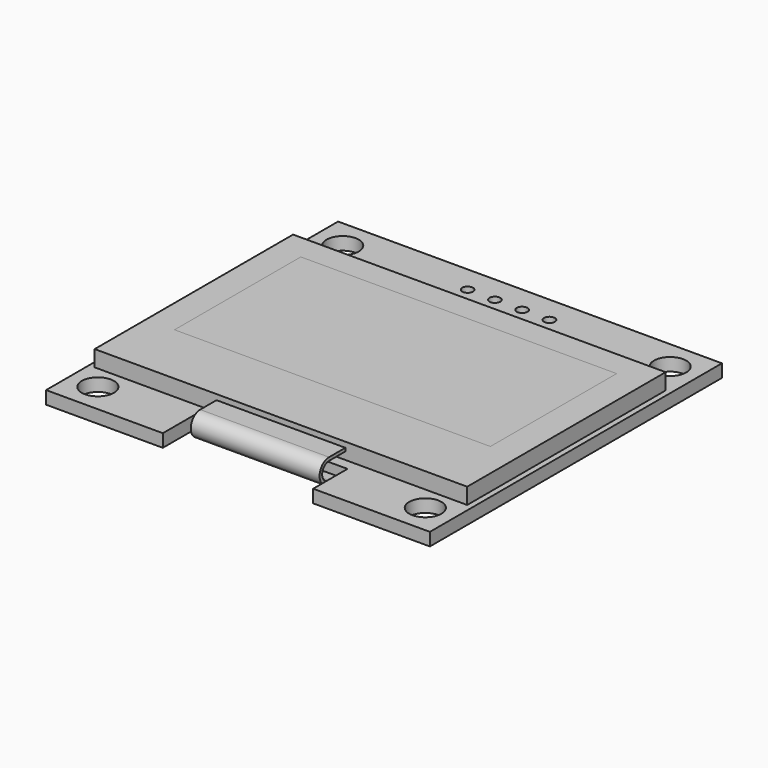
from build123d import *

# Parameters (mm, degrees)
F0_R     = 1.5
F0_R_2   = 0.5
F1_DEPTH = 1.2
F2_W     = 34.7
F2_H     = 23.1
F2_W_2   = 29.42
F2_H_2   = 14.7
F3_DEPTH = 1.5
F4_DEPTH = 1.5
F6_DEPTH = 6
F7_W     = 0.762
F7_H     = 1.524
F7_W_2   = 1.65
F7_H_2   = 3
F7_W_3   = 1.524
F7_H_3   = 0.762
F8_DEPTH = 0.9


with BuildPart() as f1:
    # F0 (on Top) → F1 (new body)
    with BuildSketch(Plane.XY):
        Polygon((17.875, 0), (17.875, 34), (-17.875, 34), (-17.875, 0), (-7, 0), (-7, 4), (7, 4), (7, 0), align=None)
        with Locations((-15.25, 2.75)):
            Circle(F0_R, mode=Mode.SUBTRACT)
        with Locations((15.25, 2.75)):
            Circle(F0_R, mode=Mode.SUBTRACT)
        with Locations((-15.25, 31.25)):
            Circle(F0_R, mode=Mode.SUBTRACT)
        with Locations((-3.81, 31.5)):
            Circle(F0_R_2, mode=Mode.SUBTRACT)
        with Locations((-1.27, 31.5)):
            Circle(F0_R_2, mode=Mode.SUBTRACT)
        with Locations((1.27, 31.5)):
            Circle(F0_R_2, mode=Mode.SUBTRACT)
        with Locations((3.81, 31.5)):
            Circle(F0_R_2, mode=Mode.SUBTRACT)
        with Locations((15.25, 31.25)):
            Circle(F0_R, mode=Mode.SUBTRACT)
    extrude(amount=-F1_DEPTH)

    # F7 (on face) → F8 (join)
    with BuildSketch(Plane(origin=(0, 0, -1.2), x_dir=(1, 0, 0), z_dir=(0, 0, -1))):
        with Locations((15.194, -16.962)):
            Rectangle(F7_W, F7_H)
        with Locations((13.1723636364, -16.962)):
            Rectangle(F7_W, F7_H)
        with Locations((11.1507272727, -16.962)):
            Rectangle(F7_W, F7_H)
        with Locations((9.1290909091, -16.962)):
            Rectangle(F7_W, F7_H)
        with Locations((7.1074545455, -16.962)):
            Rectangle(F7_W, F7_H)
        with Locations((5.0858181818, -16.962)):
            Rectangle(F7_W, F7_H)
        with Locations((3.0641818182, -16.962)):
            Rectangle(F7_W, F7_H)
        with Locations((1.0425454545, -16.962)):
            Rectangle(F7_W, F7_H)
        with Locations((-0.9790909091, -16.962)):
            Rectangle(F7_W, F7_H)
        with Locations((-3.0007272727, -16.962)):
            Rectangle(F7_W, F7_H)
        with Locations((-5.0223636364, -16.962)):
            Rectangle(F7_W, F7_H)
        with Locations((-7.044, -16.962)):
            Rectangle(F7_W, F7_H)
        with Locations((-10.082, -16.962)):
            Rectangle(F7_W, F7_H)
        with Locations((-12.544, -16.962)):
            Rectangle(F7_W, F7_H)
        with Locations((-8.15, -22.5)):
            Rectangle(F7_W_2, F7_H_2)
        with Locations((-7.413, -26.219)):
            Rectangle(F7_W_3, F7_H_3)
        with Locations((2.613, -23.219)):
            Rectangle(F7_W_3, F7_H_3)
    extrude(amount=F8_DEPTH)


with BuildPart() as f3:
    # F2 (on Top) → F3 (new body)
    with BuildSketch(Plane.XY):
        with Locations((0, 16.55)):
            Rectangle(F2_W, F2_H)
        with Locations((0, 18.35)):
            Rectangle(F2_W_2, F2_H_2, mode=Mode.SUBTRACT)
    extrude(amount=F3_DEPTH)

    # F5 (on Right) → F6 (join, symmetric)
    with BuildSketch(Plane.YZ):
        with BuildLine():
            Line((5, 1), (3.1, 1))
            ThreePointArc((3.1, 1), (2, -0.1), (3.1, -1.2))
            Line((3.1, -1.2), (4, -1.2))
            Line((4, -1.2), (4, -0.9))
            Line((4, -0.9), (3.1, -0.9))
            ThreePointArc((3.1, -0.9), (2.3, -0.1), (3.1, 0.7))
            Line((3.1, 0.7), (5, 0.7))
            Line((5, 0.7), (5, 1))
        make_face()
    extrude(amount=F6_DEPTH, both=True)


with BuildPart() as f4:
    # F2 (on Top) → F4 (new body, through all)
    with BuildSketch(Plane.XY):
        with Locations((0, 18.35)):
            Rectangle(F2_W_2, F2_H_2)
    extrude(amount=F4_DEPTH)


solid = Compound([f1.part, f3.part, f4.part])
